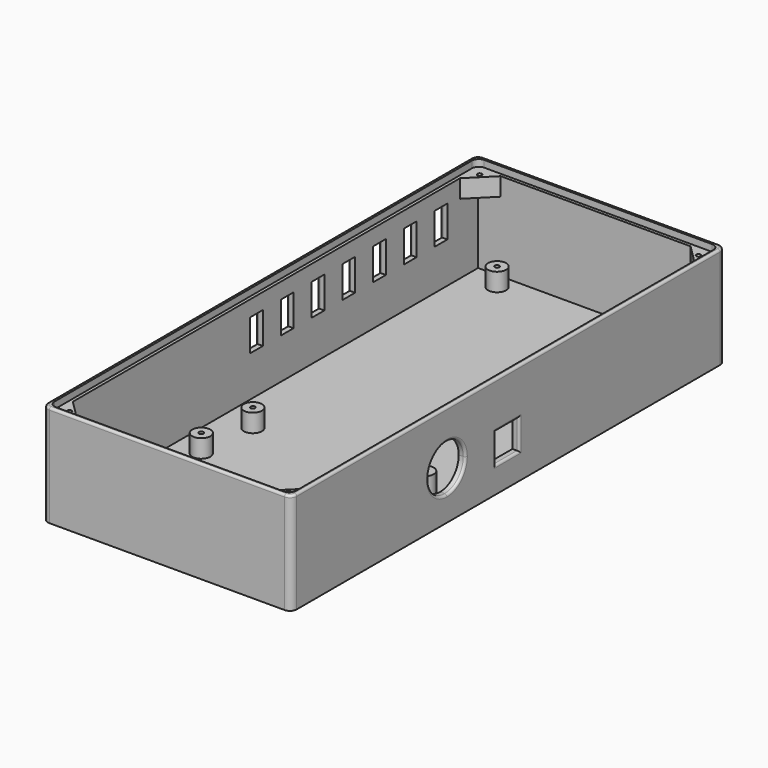
from build123d import *

# Parameters (mm, degrees)
F0_W      = 110
F0_H      = 240
F1_DEPTH  = 45
F2_W      = 104
F2_H      = 234
F3_DEPTH  = 42
F4_W      = 106.8
F4_H      = 236.8
F4_W_2    = 104
F4_H_2    = 234
F5_DEPTH  = 3
F6_R      = 4
F6_R_2    = 1
F7_DEPTH  = 8
F8_W      = 13
F8_H      = 13
F9_DEPTH  = 3
F10_W     = 7
F10_H     = 14
F11_DEPTH = 3
F12_R     = 3
F13_R     = 3
F15_DEPTH = 8
F17_DEPTH = 3
F18_D     = 2
F18_DEPTH = 6
F18_TIP   = 0.600860619
F19_R     = 1


# Not quite as in the source:
# - a feature names something its author has since deleted; it is built from what else it names


with BuildPart() as f1:
    # F0 (on Top) → F1 (new body)
    with BuildSketch(Plane.XY):
        Rectangle(F0_W, F0_H)
    extrude(amount=F1_DEPTH)

    # F2 (on face) → F3 (cut, through all)
    with BuildSketch(Plane.XY.offset(45)):
        Rectangle(F2_W, F2_H)
    extrude(amount=-F3_DEPTH, mode=Mode.SUBTRACT)

    # F4 (on face) → F5 (cut)
    with BuildSketch(Plane.XY.offset(45)):
        Rectangle(F4_W, F4_H)
        Rectangle(F4_W_2, F4_H_2, mode=Mode.SUBTRACT)
    extrude(amount=-F5_DEPTH, mode=Mode.SUBTRACT)

    # F6 (on face) → F7 (join)
    with BuildSketch(Plane.XY.offset(3)):
        with Locations((-38, 110)):
            Circle(F6_R)
        with Locations((-38, 110)):
            Circle(F6_R_2, mode=Mode.SUBTRACT)
        with Locations((38, 110)):
            Circle(F6_R)
        with Locations((38, 110)):
            Circle(F6_R_2, mode=Mode.SUBTRACT)
        with Locations((-38, -25)):
            Circle(F6_R)
        with Locations((-38, -25)):
            Circle(F6_R_2, mode=Mode.SUBTRACT)
        with Locations((38, -25)):
            Circle(F6_R)
        with Locations((38, -25)):
            Circle(F6_R_2, mode=Mode.SUBTRACT)
        with Locations((-40, -51)):
            Circle(F6_R)
        with Locations((-40, -51)):
            Circle(F6_R_2, mode=Mode.SUBTRACT)
        with Locations((40, -51)):
            Circle(F6_R)
        with Locations((40, -51)):
            Circle(F6_R_2, mode=Mode.SUBTRACT)
        with Locations((-40, -109)):
            Circle(F6_R)
        with Locations((-40, -109)):
            Circle(F6_R_2, mode=Mode.SUBTRACT)
        with Locations((40, -109)):
            Circle(F6_R)
        with Locations((40, -109)):
            Circle(F6_R_2, mode=Mode.SUBTRACT)
    extrude(amount=F7_DEPTH)

    # F8 (on face) → F9 (cut, through all)
    with BuildSketch(Plane.YZ.offset(55)):
        with Locations((-0.5, 18)):
            Rectangle(F8_W, F8_H)
    extrude(amount=-F9_DEPTH, mode=Mode.SUBTRACT)

    # F10 (on face) → F11 (cut, through all)
    with BuildSketch(Plane(origin=(-55, 0, 0), x_dir=(0, -1, 0), z_dir=(-1, 0, 0))):
        with Locations((-62.5, 28)):
            Rectangle(F10_W, F10_H)
        with Locations((-45.5, 28)):
            Rectangle(F10_W, F10_H)
        with Locations((-28.5, 28)):
            Rectangle(F10_W, F10_H)
        with Locations((-11.5, 28)):
            Rectangle(F10_W, F10_H)
        with Locations((5.5, 28)):
            Rectangle(F10_W, F10_H)
        with Locations((-79.5, 28)):
            Rectangle(F10_W, F10_H)
        with Locations((-96.5, 28)):
            Rectangle(F10_W, F10_H)
    extrude(amount=-F11_DEPTH, mode=Mode.SUBTRACT)

    # F12
    f12_edges = [f1.edges().sort_by_distance(p)[0] for p in [
        (-55, -120, 22.5),
        (55, -120, 22.5),
        (-55, 120, 22.5),
        (55, 120, 22.5),
    ]]
    fillet(f12_edges, radius=F12_R)

    # F13
    f13_edges = [f1.edges().sort_by_distance(p)[0] for p in [
        (-53.4, 118.4, 43.5),
        (53.4, 118.4, 43.5),
        (53.4, -118.4, 43.5),
        (-53.4, -118.4, 43.5),
    ]]
    fillet(f13_edges, radius=F13_R)

    # F14 (on face) → F15 (join)
    with BuildSketch(Plane.XY.offset(42)):
        Polygon((-42, 117), (-52, 117), (-52, 107), align=None)
        Polygon((52, 107), (52, 117), (42, 117), align=None)
        Polygon((42, -117), (52, -117), (52, -107), align=None)
        Polygon((-52, -107), (-52, -117), (-42, -117), align=None)
    extrude(amount=-F15_DEPTH)

    # F16 (on face) → F17 (cut, through all)
    with BuildSketch(Plane.YZ.offset(55)):
        with BuildLine():
            ThreePointArc((-33.9475087821, 11), (-26.699664275, 14.0021554928), (-23.6975087821, 21.25))
            ThreePointArc((-23.6975087821, 21.25), (-41.1953532893, 28.4978445072), (-33.9475087821, 11))
        make_face()
    extrude(amount=-F17_DEPTH, mode=Mode.SUBTRACT)

    # F18
    with Locations(Plane.XY.offset(42)):
        with Locations((48.4, 113.4), (-48.4, 113.4), (-48.4, -113.4), (48.4, -113.4)):
            Hole(F18_D / 2, depth=F18_DEPTH)
            with Locations((0, 0, -(F18_DEPTH + F18_TIP / 2))):  # 118° drill point
                Cone(0, F18_D / 2, F18_TIP, mode=Mode.SUBTRACT)

    # F19
    f19_edges = [f1.edges().sort_by_distance(p)[0] for p in [
        (0, -120, 45),
        (55, -33.947509, 31.5),
        (55, -7, 18),
        (55, -0.5, 11.5),
        (55, 6, 18),
        (55, -0.5, 24.5),
        (-55, 100, 28),
        (-55, 93, 28),
        (-55, 96.5, 21),
        (-55, 96.5, 35),
        (-55, 79.5, 35),
        (-55, 83, 28),
        (-55, 79.5, 21),
        (-55, 76, 28),
        (-55, 62.5, 35),
        (-55, 66, 28),
        (-55, 62.5, 21),
        (-55, 59, 28),
        (-55, 45.5, 35),
        (-55, 42, 28),
        (-55, 49, 28),
        (-55, 45.5, 21),
        (-55, 32, 28),
        (-55, 28.5, 21),
        (-55, 28.5, 35),
        (-55, 25, 28),
        (-55, 15, 28),
        (-55, 11.5, 21),
        (-55, 11.5, 35),
        (-55, 8, 28),
        (-55, -5.5, 35),
        (-55, -2, 28),
        (-55, -9, 28),
        (-55, -5.5, 21),
    ]]
    fillet(f19_edges, radius=F19_R)


solid = f1.part
